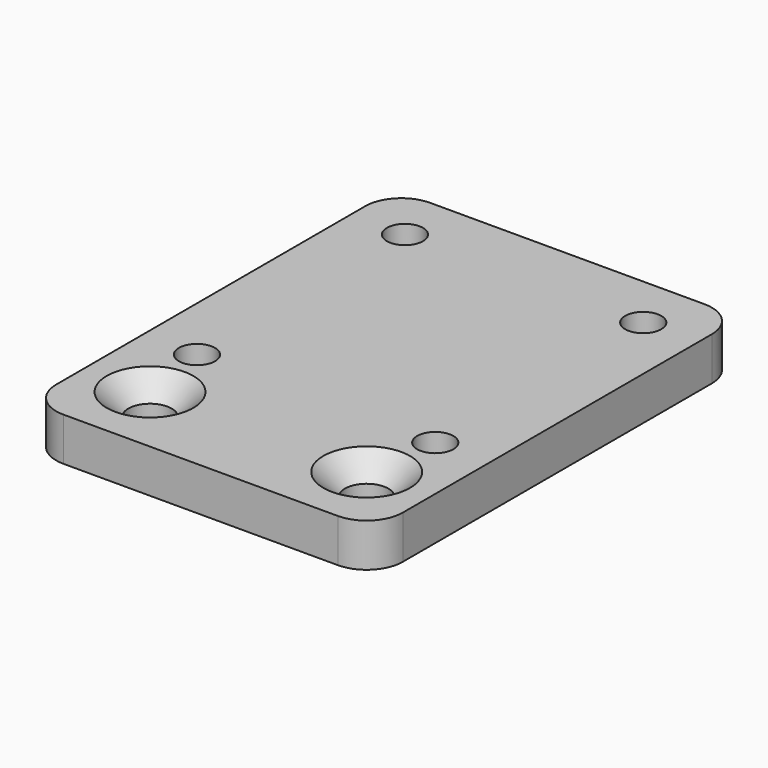
from build123d import *

# Parameters (mm, degrees)
F0_W           = 48
F0_H           = 63.5
F1_DEPTH       = 6
F2_R           = 5
F3_D           = 5
F4_D           = 6
F4_CSINK_D     = 12
F4_CSINK_ANGLE = 90


# Not quite as in the source:
# - a feature names something its author has since deleted; it is built from what else it names


with BuildPart() as f1:
    # F0 (on Top) → F1 (new body)
    with BuildSketch(Plane.XY):
        with Locations((0, 12.75)):
            Rectangle(F0_W, F0_H)
    extrude(amount=-F1_DEPTH)

    # F2
    f2_edges = [f1.edges().sort_by_distance(p)[0] for p in [
        (-24, -19, -3),
        (-24, 44.5, -3),
        (24, -19, -3),
        (24, 44.5, -3),
    ]]
    fillet(f2_edges, radius=F2_R)

    # F3 (through all)
    with Locations(Plane.XY):
        with Locations((16.5, 1), (-16.5, 1), (16.5, 37), (-16.5, 37)):
            Hole(F3_D / 2)

    # F4 (through all)
    with Locations(Plane.XY):
        with Locations((15, -9), (-15, -9)):
            CounterSinkHole(F4_D / 2, F4_CSINK_D / 2, counter_sink_angle=F4_CSINK_ANGLE)


solid = f1.part
